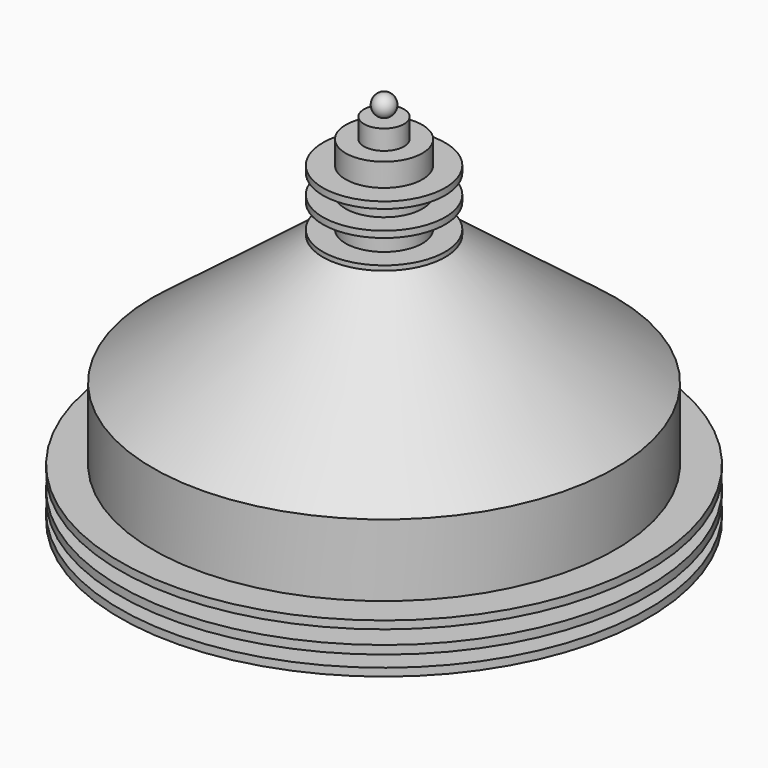
from build123d import *

# Parameters (mm, degrees)
F0_W   = 11.6114281118
F0_H   = 11.429999955
F0_W_2 = 22.2317185253
F0_H_2 = 11.1170867458
F0_H_3 = 13.9705389738
F2_T   = 2.54


# Not quite as in the source:
# - a shell that OpenCascade refuses in one call is made with other operations: the cavity is built on its own and cut out


with BuildPart() as f1:
    # F0 (on Front) → F1 (revolve)
    with BuildSketch(Plane.XZ):
        Polygon((0, -187.8297179937), (0, -41.9409945607), (-35.0329726934, -41.9409945607), (-133.9662224054, -117.5266578425), (-133.9662224054, -159.1617912054), (-152.9530584812, -159.1617912054), (-152.9530584812, -163.6997163296), (-133.9662224054, -163.6997163296), (-133.9662224054, -171.6825813055), (-152.9530584812, -171.6825813055), (-152.9530584812, -176.581159234), (-133.9662224054, -176.581159234), (-133.9662224054, -183.2940131426), (-152.9530584812, -183.2940131426), (-152.9530584812, -187.8297179937), align=None)
        with Locations((-5.8057140559, 12.5185712241)):
            Rectangle(F0_W, F0_H)
        Polygon((0, -6.5624886192), (0, 6.8035712466), (-11.6114281118, 6.8035712466), (-22.2317185253, 6.8035712466), (-22.2317185253, -6.5624886192), align=None)
        Polygon((0, -10.4182204232), (0, -6.5624886192), (-22.2317185253, -6.5624886192), (-35.4292169213, -6.5624886192), (-35.4292169213, -10.4182204232), (-22.2317185253, -10.4182204232), align=None)
        with Locations((-11.1158592626, -15.9767637961)):
            Rectangle(F0_W_2, F0_H_2)
        Polygon((0, -25.2490267158), (0, -21.535307169), (-22.2317185253, -21.535307169), (-35.4292169213, -21.535307169), (-35.4292169213, -25.2490267158), (-22.2317185253, -25.2490267158), align=None)
        with Locations((-11.1158592626, -32.2342962027)):
            Rectangle(F0_W_2, F0_H_3)
        Polygon((0, -41.9409945607), (0, -39.2195656896), (-22.2317185253, -39.2195656896), (-35.4292169213, -39.2195656896), (-35.4292169213, -41.9409945607), (-35.0329726934, -41.9409945607), align=None)
    revolve(axis=Axis((0, 0, -78.7202166393), (0, 0, -1)))

    # F2: shell of thickness 2.54, made by hand


with BuildPart() as f1b:
    # F0 (on Front) → F1, piece 2 (revolve)
    with BuildSketch(Plane.XZ):
        with BuildLine():
            Line((0, 18.2335712016), (0, 30.3892847151))
            ThreePointArc((0, 30.3892847151), (-6.0778567567, 24.3114279583), (0, 18.2335712016))
        make_face()
    revolve(axis=Axis((0, 0, -78.7202166393), (0, 0, -1)))


with BuildPart() as f2_core1:
    # F2_t2: copy of F1
    add(f1.part)

    # the walls: a layer under each face that stays
    f2_faces = [f2_core1.faces().sort_by_distance(p)[0] for p in [
        (0, 0, 18.2335712016),
        (11.6114281118, 0, 12.5185712241),
        (-14.8211456835, -14.8211456835, 6.8035712466),
        (22.2317185253, 0, 0.1205413137),
        (-23.6194779476, -23.6194779476, -6.5624886192),
        (35.4292169213, 0, -8.4903545212),
        (23.6194779476, -23.6194779476, -10.4182204232),
        (22.2317185253, 0, -15.9767637961),
        (-23.6194779476, -23.6194779476, -21.535307169),
        (35.4292169213, 0, -23.3921669424),
        (23.6194779476, -23.6194779476, -25.2490267158),
        (22.2317185253, 0, -32.2342962027),
        (-23.6194779476, -23.6194779476, -39.2195656896),
        (35.4292169213, 0, -40.5802801251),
        (-31.0005648062, -17.058511851, -41.9409945607),
        (84.4995975494, 0, -79.7338262016),
        (133.9662224054, 0, -138.344224524),
        (-101.9687056541, -101.9687056541, -159.1617912054),
        (152.9530584812, 0, -161.4307537675),
        (101.9687056541, -101.9687056541, -163.6997163296),
        (133.9662224054, 0, -167.6911488175),
        (-101.9687056541, -101.9687056541, -171.6825813055),
        (152.9530584812, 0, -174.1318702698),
        (101.9687056541, -101.9687056541, -176.581159234),
        (133.9662224054, 0, -179.9375861883),
        (-101.9687056541, -101.9687056541, -183.2940131426),
        (152.9530584812, 0, -185.5618655682),
    ]]
    thicken(f2_faces, amount=-F2_T, mode=Mode.SUBTRACT)

    # F2_s3 → F2_t4 (revolve, cut)
    with BuildSketch(Plane.XZ):
        Polygon((-11.6368281118, 6.8289712466), (-9.0714281118, 6.8035712466), (-9.0714281118, 4.2635712466), (-11.6114281118, 4.2635712466), align=None)
    revolve(axis=Axis((0, 0, 6.8035712466), (0, 0, -1)), mode=Mode.SUBTRACT)

    # F2_s5 → F2_t6 (revolve, cut)
    with BuildSketch(Plane.XZ):
        Polygon((-22.2571185253, -6.5370886192), (-19.6917185253, -6.5624886192), (-19.6917185253, -9.1024886192), (-22.2317185253, -9.1024886192), align=None)
    revolve(axis=Axis((0, 0, -6.5624886192), (0, 0, -1)), mode=Mode.SUBTRACT)

    # F2_s7 → F2_t8 (revolve, cut)
    with BuildSketch(Plane.XZ):
        Polygon((-22.2571185253, -10.4436204232), (-22.2317185253, -7.8782204232), (-19.6917185253, -7.8782204232), (-19.6917185253, -10.4182204232), align=None)
    revolve(axis=Axis((0, 0, -10.4182204232), (0, 0, -1)), mode=Mode.SUBTRACT)

    # F2_s9 → F2_t10 (revolve, cut)
    with BuildSketch(Plane.XZ):
        Polygon((-22.2571185253, -21.509907169), (-19.6917185253, -21.535307169), (-19.6917185253, -24.075307169), (-22.2317185253, -24.075307169), align=None)
    revolve(axis=Axis((0, 0, -21.535307169), (0, 0, -1)), mode=Mode.SUBTRACT)

    # F2_s11 → F2_t12 (revolve, cut)
    with BuildSketch(Plane.XZ):
        Polygon((-22.2571185253, -25.2744267158), (-22.2317185253, -22.7090267158), (-19.6917185253, -22.7090267158), (-19.6917185253, -25.2490267158), align=None)
    revolve(axis=Axis((0, 0, -25.2490267158), (0, 0, -1)), mode=Mode.SUBTRACT)

    # F2_s13 → F2_t14 (revolve, cut)
    with BuildSketch(Plane.XZ):
        Polygon((-22.2571185253, -39.1941656896), (-19.6917185253, -39.2195656896), (-19.6917185253, -41.7595656896), (-22.2317185253, -41.7595656896), align=None)
    revolve(axis=Axis((0, 0, -39.2195656896), (0, 0, -1)), mode=Mode.SUBTRACT)

    # F2_s15 → F2_t16 (revolve, cut)
    with BuildSketch(Plane.XZ):
        Polygon((-35.0483930197, -41.946211064), (-35.0329726934, -39.4009945607), (-27.5245659384, -39.4009945607), (-33.4909400706, -43.9593442307), align=None)
    revolve(axis=Axis((0, 0, -41.9409945607), (0, 0, -1)), mode=Mode.SUBTRACT)

    # F2_s17 → F2_t18 (revolve, cut)
    with BuildSketch(Plane.XZ):
        Polygon((-133.9916224054, -159.1363912054), (-131.4262224054, -159.1617912054), (-131.4262224054, -161.7017912054), (-133.9662224054, -161.7017912054), align=None)
    revolve(axis=Axis((0, 0, -159.1617912054), (0, 0, -1)), mode=Mode.SUBTRACT)

    # F2_s19 → F2_t20 (revolve, cut)
    with BuildSketch(Plane.XZ):
        Polygon((-133.9916224054, -163.7251163296), (-133.9662224054, -161.1597163296), (-131.4262224054, -161.1597163296), (-131.4262224054, -163.6997163296), align=None)
    revolve(axis=Axis((0, 0, -163.6997163296), (0, 0, -1)), mode=Mode.SUBTRACT)

    # F2_s21 → F2_t22 (revolve, cut)
    with BuildSketch(Plane.XZ):
        Polygon((-133.9916224054, -171.6571813055), (-131.4262224054, -171.6825813055), (-131.4262224054, -174.2225813055), (-133.9662224054, -174.2225813055), align=None)
    revolve(axis=Axis((0, 0, -171.6825813055), (0, 0, -1)), mode=Mode.SUBTRACT)

    # F2_s23 → F2_t24 (revolve, cut)
    with BuildSketch(Plane.XZ):
        Polygon((-133.9916224054, -176.606559234), (-133.9662224054, -174.041159234), (-131.4262224054, -174.041159234), (-131.4262224054, -176.581159234), align=None)
    revolve(axis=Axis((0, 0, -176.581159234), (0, 0, -1)), mode=Mode.SUBTRACT)

    # F2_s25 → F2_t26 (revolve, cut)
    with BuildSketch(Plane.XZ):
        Polygon((-133.9916224054, -183.2686131426), (-131.4262224054, -183.2940131426), (-131.4262224054, -185.8340131426), (-133.9662224054, -185.8340131426), align=None)
    revolve(axis=Axis((0, 0, -183.2940131426), (0, 0, -1)), mode=Mode.SUBTRACT)


with BuildPart() as f1_1:
    add(f1.part)

    # what is left inside the walls is the cavity
    f2_cavity = [f2_core1.part.solids().sort_by_distance(p)[0] for p in [
        (0, -50.137686, -187.804318),
    ]]
    add(f2_cavity, mode=Mode.SUBTRACT)


solid = Compound([f1b.part, f1_1.part])
